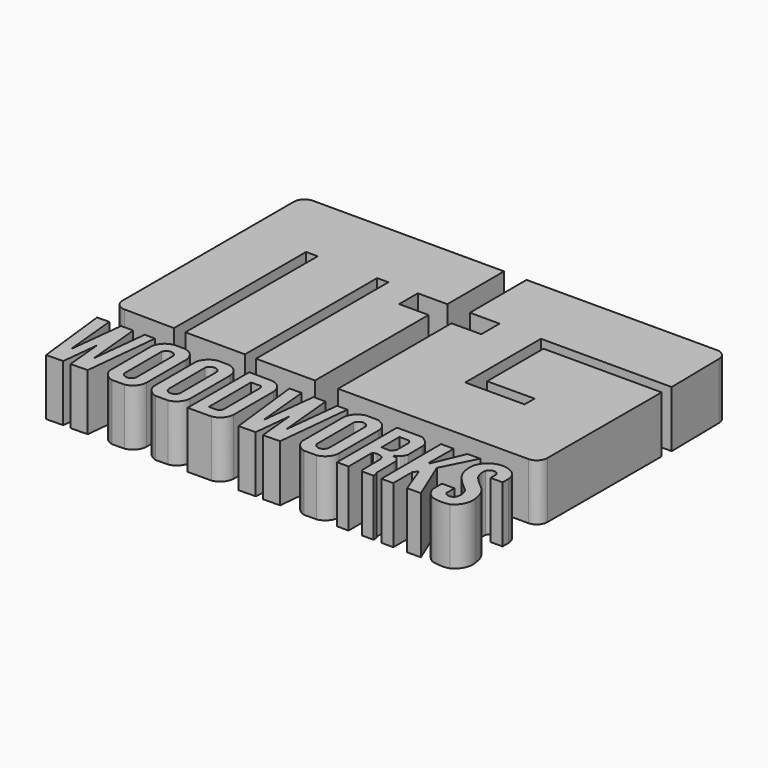
from build123d import *

# Parameters (mm, degrees)
F1_DEPTH = 12.7


# Not quite as in the source:
# - ends of sketch curves that miss each other by under 0.0002 mm in the source are joined


with BuildPart() as f1:
    # F0 (on Top) → F1 (new body)
    with BuildSketch(Plane.XY):
        with BuildLine():
            Line((-2.536317, 21.6905332), (-2.5611328, 37.6696224))
            Line((-2.5611328, 37.6696224), (-45.544359, 37.6696224))
            ThreePointArc((-45.544359, 37.6696224), (-47.2281570227, 36.9721704227), (-47.925609, 35.2883724))
            Line((-47.925609, 35.2883724), (-47.925609, -12.8909064))
            ThreePointArc((-47.925609, -12.8909064), (-47.2392470168, -14.5635409008), (-45.575829537, -15.271948434))
            Line((-45.575829537, -15.271948434), (-34.336101, -15.4204924))
            Line((-34.336101, -15.4204924), (-34.315146, 21.7128852))
            Line((-34.315146, 21.7128852), (-31.6947042, 21.7128852))
            Line((-31.6947042, 21.7128852), (-31.7876936, -15.4014678))
            Line((-31.7876936, -15.4014678), (-18.371058, -15.4014678))
            Line((-18.371058, -15.4014678), (-18.371058, 21.7389964))
            Line((-18.371058, 21.7389964), (-15.8285942, 21.7389964))
            Line((-15.8285942, 21.7389964), (-15.8285942, -15.4928316))
            Line((-15.8285942, -15.4928316), (-2.5525984, -15.4928316))
            Line((-2.5525984, -15.4928316), (-2.5525984, 16.4305996))
            Line((-2.5525984, 16.4305996), (-9.1684094, 16.4305996))
            Line((-9.1684094, 16.4305996), (-9.1684094, 21.6905332))
            Line((-9.1684094, 21.6905332), (-2.536317, 21.6905332))
        make_face()
    extrude(amount=F1_DEPTH)


with BuildPart() as f1b:
    # F0 (on Top) → F1, piece 2 (new body)
    with BuildSketch(Plane.XY):
        with BuildLine():
            Line((45.3263762, 37.6347736), (2.5456388, 37.5991628))
            Line((2.5456388, 37.5991628), (2.5893776, 21.6360502))
            Line((2.5893776, 21.6360502), (9.25957, 21.6360502))
            Line((9.25957, 21.6360502), (9.25957, 16.490442))
            Line((9.25957, 16.490442), (2.572131, 16.452342))
            Line((2.572131, 16.452342), (2.572131, -15.4098498))
            Line((2.572131, -15.4098498), (45.356907, -15.4098498))
            ThreePointArc((45.356907, -15.4098498), (47.0389799334, -14.7141211464), (47.7381520062, -13.0334765898))
            Line((47.7381520062, -13.0334765898), (47.8035112, 19.010757))
            Line((47.8035112, 19.010757), (21.2254084, 19.010757))
            Line((21.2254084, 19.010757), (21.2254084, 3.1541466))
            Line((21.2254084, 3.1541466), (31.8709294, 3.2285686))
            Line((31.8709294, 3.2285686), (31.8709294, 0.3996944))
            Line((31.8709294, 0.3996944), (18.5200798, 0.3996944))
            Line((18.5200798, 0.3996944), (18.5200798, 21.6888822))
            Line((18.5200798, 21.6888822), (47.9255836, 21.6888822))
            Line((47.9255836, 21.6888822), (47.7093026, 35.291395))
            ThreePointArc((47.7093026, 35.291395), (46.9980060234, 36.9513531076), (45.3263762, 37.6347736))
        make_face()
    extrude(amount=F1_DEPTH)


with BuildPart() as f1c:
    # F0 (on Top) → F1, piece 3 (new body)
    with BuildSketch(Plane.XY):
        Polygon((-44.7095626, -20.636865), (-47.4261434, -20.673441), (-45.4905872, -37.4233948), (-41.6939222, -37.3489474), (-40.8006042, -29.0111942), (-39.9817082, -37.4233948), (-36.1850686, -37.3489474), (-34.4728292, -20.5989936), (-36.7693448, -20.5808072), (-38.1679196, -33.2048104), (-39.3644882, -20.5760828), (-42.086657, -20.5760828), (-43.497754, -32.9671172), align=None)
    extrude(amount=F1_DEPTH)


with BuildPart() as f1d:
    # F0 (on Top) → F1, piece 4 (new body)
    with BuildSketch(Plane.XY):
        with BuildLine():
            ThreePointArc((-30.2710578131, -20.3485617265), (-32.12595589, -21.2621265704), (-33.0999267378, -23.0860312794))
            Line((-33.0999267378, -23.0860312794), (-33.0999084, -34.9780606))
            ThreePointArc((-33.0999084, -34.9780606), (-32.1862490905, -36.6588109238), (-30.5363625494, -37.6271026097))
            Line((-30.5363625494, -37.6271026097), (-27.7310596, -37.6025918))
            ThreePointArc((-27.7310596, -37.6025918), (-25.9105020583, -36.5706907109), (-25.1482772788, -34.621774272))
            Line((-25.1482772788, -34.621774272), (-25.1482606, -23.4615736))
            ThreePointArc((-25.1482606, -23.4615736), (-25.982709746, -21.4149466319), (-27.9292558062, -20.3680822415))
            Line((-27.9292558062, -20.3680822415), (-30.2710578131, -20.3485617265))
        make_face()
        with BuildLine():
            Line((-30.413833, -34.051113), (-30.4320702, -23.8051848))
            ThreePointArc((-30.4320702, -23.8051848), (-29.1470080176, -22.7652283211), (-27.8315931927, -23.7665007022))
            Line((-27.8315931927, -23.7665007022), (-27.8011128, -34.0119462))
            ThreePointArc((-27.8011128, -34.0119462), (-29.089713326, -35.2161905196), (-30.413833, -34.051113))
        make_face(mode=Mode.SUBTRACT)
    extrude(amount=F1_DEPTH)


with BuildPart() as f1e:
    # F0 (on Top) → F1, piece 5 (new body)
    with BuildSketch(Plane.XY):
        with BuildLine():
            ThreePointArc((-20.4964302764, -20.2723114663), (-22.351335001, -21.1858857482), (-23.3252999912, -23.0098050731))
            Line((-23.3252999912, -23.0098050731), (-23.3252772, -34.9018352))
            ThreePointArc((-23.3252772, -34.9018352), (-22.4116093547, -36.5825943442), (-20.7617076236, -37.5508835121))
            Line((-20.7617076236, -37.5508835121), (-17.956403, -37.5263664))
            ThreePointArc((-17.956403, -37.5263664), (-16.1358457214, -36.4944656146), (-15.3736207042, -34.5455496753))
            Line((-15.3736207042, -34.5455496753), (-15.3736294, -23.3853482))
            ThreePointArc((-15.3736294, -23.3853482), (-16.208043765, -21.3387062672), (-18.1545954939, -20.2918319962))
            Line((-18.1545954939, -20.2918319962), (-20.4964302764, -20.2723114663))
        make_face()
        with BuildLine():
            Line((-20.6391764, -33.9748876), (-20.6574136, -23.7289594))
            ThreePointArc((-20.6574136, -23.7289594), (-19.3723739853, -22.689002879), (-18.0569619927, -23.6902753022))
            Line((-18.0569619927, -23.6902753022), (-18.0264562, -33.9356954))
            ThreePointArc((-18.0264562, -33.9356954), (-19.3150441078, -35.1399395303), (-20.6391764, -33.9748876))
        make_face(mode=Mode.SUBTRACT)
    extrude(amount=F1_DEPTH)


with BuildPart() as f1f:
    # F0 (on Top) → F1, piece 6 (new body)
    with BuildSketch(Plane.XY):
        with BuildLine():
            ThreePointArc((12.9104371236, -20.2723114663), (11.055532399, -21.1858857482), (10.0815674088, -23.0098050731))
            Line((10.0815674088, -23.0098050731), (10.0815902, -34.9018352))
            ThreePointArc((10.0815902, -34.9018352), (10.9952580453, -36.5825943442), (12.6451597764, -37.5508835121))
            Line((12.6451597764, -37.5508835121), (15.4504644, -37.5263664))
            ThreePointArc((15.4504644, -37.5263664), (17.2710216786, -36.4944656146), (18.0332466958, -34.5455496753))
            Line((18.0332466958, -34.5455496753), (18.033238, -23.3853482))
            ThreePointArc((18.033238, -23.3853482), (17.198823635, -21.3387062672), (15.2522719061, -20.2918319962))
            Line((15.2522719061, -20.2918319962), (12.9104371236, -20.2723114663))
        make_face()
        with BuildLine():
            Line((12.767691, -33.9748876), (12.7494538, -23.7289594))
            ThreePointArc((12.7494538, -23.7289594), (14.0344934147, -22.689002879), (15.3499054073, -23.6902753022))
            Line((15.3499054073, -23.6902753022), (15.3804112, -33.9356954))
            ThreePointArc((15.3804112, -33.9356954), (14.0918232922, -35.1399395303), (12.767691, -33.9748876))
        make_face(mode=Mode.SUBTRACT)
    extrude(amount=F1_DEPTH)


with BuildPart() as f1g:
    # F0 (on Top) → F1, piece 7 (new body)
    with BuildSketch(Plane.XY):
        Polygon((-1.4388338, -20.636865), (-4.1554146, -20.673441), (-2.2198584, -37.4233948), (1.5768066, -37.3489474), (2.4701246, -29.0111942), (3.2890206, -37.4233948), (7.0856856, -37.3489474), (8.7978996, -20.5989936), (6.501384, -20.5808072), (5.1028346, -33.2048104), (3.9062406, -20.5760828), (1.1840718, -20.5760828), (-0.2270252, -32.9671172), align=None)
    extrude(amount=F1_DEPTH)


with BuildPart() as f1h:
    # F0 (on Top) → F1, piece 8 (new body)
    with BuildSketch(Plane.XY):
        with BuildLine():
            Line((-8.3665568, -20.2918568), (-13.5372348, -20.248753))
            Line((-13.5372348, -20.248753), (-13.5372348, -37.5732548))
            Line((-13.5372348, -37.5732548), (-8.1683606, -37.5263664))
            ThreePointArc((-8.1683606, -37.5263664), (-6.3478033214, -36.4944656146), (-5.5855783042, -34.5455496753))
            Line((-5.5855783042, -34.5455496753), (-5.585587, -23.3853482))
            ThreePointArc((-5.585587, -23.3853482), (-6.420001365, -21.3387062672), (-8.3665568, -20.2918568))
        make_face()
        with BuildLine():
            Line((-10.8493814, -34.9561658), (-10.870565, -23.0604568))
            Line((-10.870565, -23.0604568), (-8.6387432, -23.0604568))
            ThreePointArc((-8.6387432, -23.0604568), (-8.4100565801, -23.3496634959), (-8.2689195927, -23.6902753022))
            Line((-8.2689195927, -23.6902753022), (-8.2384138, -33.9356954))
            ThreePointArc((-8.2384138, -33.9356954), (-8.4336501182, -34.5233834131), (-8.8765830699, -34.9561754528))
            Line((-8.8765830699, -34.9561754528), (-10.8493814, -34.9561658))
        make_face(mode=Mode.SUBTRACT)
    extrude(amount=F1_DEPTH)


with BuildPart() as f1i:
    # F0 (on Top) → F1, piece 9 (new body)
    with BuildSketch(Plane.XY):
        Polygon((19.8892668, -20.5179168), (19.8892668, -37.3363744), (22.478873, -37.3509032), (22.4652078, -30.860111), (22.6213162, -30.5947064), (23.4175554, -30.4541936), (24.2137692, -30.5634898), (24.8850912, -30.9694072), (25.1192538, -31.734379), (25.1911866, -36.746307), (25.4659384, -37.3208296), (28.0887932, -37.3458232), (28.0513028, -36.3965998), (27.7822406, -36.185094), (27.7517606, -31.153862), (27.5992844, -30.239081), (26.9589504, -29.5072816), (26.1783576, -29.364559), (26.1783576, -29.1303964), (26.6467082, -28.9352482), (27.1540986, -28.4668722), (27.5053806, -28.096083), (27.83713, -27.3935444), (27.7981156, -23.295356), (27.6966172, -22.8465126), (27.5405088, -22.2532702), (27.0096996, -21.5351106), (26.3227566, -20.9574638), (25.6065782, -20.5179168), align=None)
        Polygon((24.2072668, -28.0706322), (22.4470214, -28.0277062), (22.4431098, -22.9810818), (24.5663466, -22.9967028), (24.8317512, -23.1840532), (25.1596144, -23.7304834), (25.1439934, -27.1182846), (24.9254264, -27.524202), (24.519509, -27.8832818), align=None, mode=Mode.SUBTRACT)
    extrude(amount=F1_DEPTH)


with BuildPart() as f1j:
    # F0 (on Top) → F1, piece 10 (new body)
    with BuildSketch(Plane.XY):
        Polygon((29.8376594, -20.560411), (29.9063156, -37.3810022), (32.5558658, -37.3624348), (32.5597774, -32.0738246), (33.293558, -31.0434228), (35.6665784, -37.3702326), (38.749986, -37.3507254), (34.9054928, -28.0810462), (38.691439, -20.5677262), (35.8422194, -20.5872334), (32.8759312, -27.534616), (32.622236, -27.534616), (32.686879, -20.5408784), align=None)
    extrude(amount=F1_DEPTH)


with BuildPart() as f1k:
    # F0 (on Top) → F1, piece 11 (new body)
    with BuildSketch(Plane.XY):
        with BuildLine():
            Line((39.3789154, -32.2001896), (39.3789154, -34.6825062))
            ThreePointArc((39.3789154, -34.6825062), (40.0290229514, -36.1759085937), (41.2239497461, -37.282723359))
            ThreePointArc((41.2239497461, -37.282723359), (43.2793077018, -37.660991127), (45.3611491688, -37.4778794294))
            ThreePointArc((45.3611491688, -37.4778794294), (47.219768062, -35.4869629879), (47.4688029965, -32.7747344446))
            ThreePointArc((47.4688029965, -32.7747344446), (46.8884969735, -30.7053849334), (45.5953463526, -28.9887809185))
            ThreePointArc((45.5953463526, -28.9887809185), (44.2366357205, -27.8576049079), (43.0123196333, -26.5821832473))
            ThreePointArc((43.0123196333, -26.5821832473), (42.3289234058, -25.1810408679), (42.3253632055, -23.6221205471))
            ThreePointArc((42.3253632055, -23.6221205471), (43.4750884405, -22.7520264357), (44.6609519713, -23.5721634455))
            Line((44.6609519713, -23.5721634455), (44.6734438, -25.1708666))
            Line((44.6734438, -25.1708666), (47.3712286, -25.1583698))
            Line((47.3712286, -25.1583698), (47.3712286, -23.472267))
            ThreePointArc((47.3712286, -23.472267), (47.1235054469, -22.3887909436), (46.5432094535, -21.4408805206))
            ThreePointArc((46.5432094535, -21.4408805206), (44.5069579511, -20.3507402941), (42.1980598999, -20.4117650875))
            ThreePointArc((42.1980598999, -20.4117650875), (40.1457165619, -21.8348360011), (39.3012785685, -24.185193693))
            ThreePointArc((39.3012785685, -24.185193693), (39.558422606, -26.1454101489), (40.3663805979, -27.9497857403))
            ThreePointArc((40.3663805979, -27.9497857403), (41.9875838504, -29.7504210155), (43.8283713407, -31.3258815952))
            ThreePointArc((43.8283713407, -31.3258815952), (44.5895599783, -32.8767072338), (44.3591707589, -34.5888315298))
            ThreePointArc((44.3591707589, -34.5888315298), (43.2359488342, -35.1082456901), (42.189095645, -34.4483179508))
            Line((42.189095645, -34.4483179508), (42.1890952, -32.2001896))
            Line((42.1890952, -32.2001896), (39.3789154, -32.2001896))
        make_face()
    extrude(amount=F1_DEPTH)


solid = Compound([f1.part, f1b.part, f1c.part, f1d.part, f1e.part, f1f.part, f1g.part, f1h.part, f1i.part, f1j.part, f1k.part])
